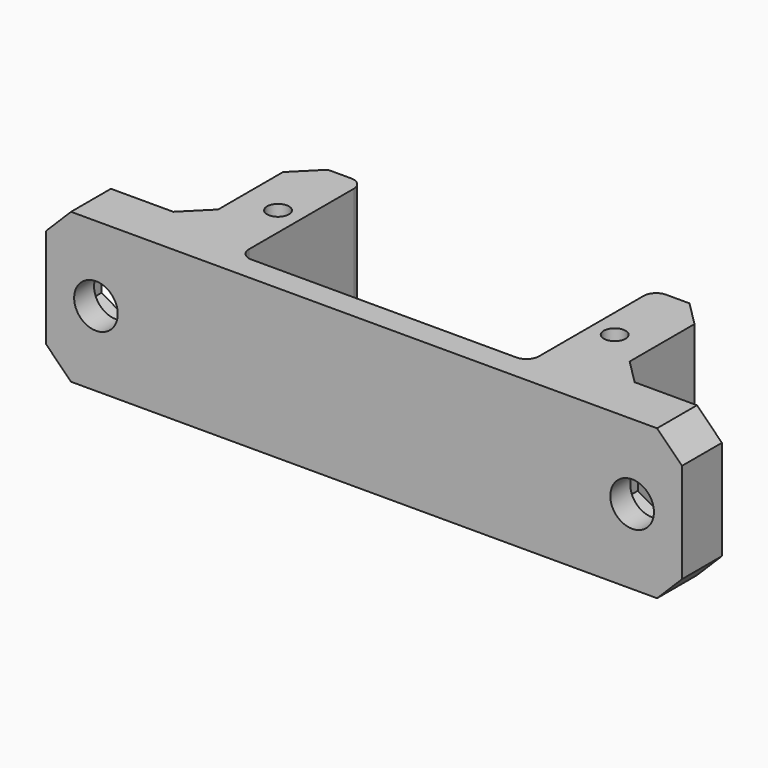
from build123d import *

# Parameters (mm, degrees)
F0_R     = 0.875
F1_DEPTH = 12
F2_SIZE  = 2
F3_R     = 1.75
F4_DEPTH = 4
F5_DEPTH = 2
F6_R     = 1


with BuildPart() as f1:
    # F0 (on Top) → F1 (new body)
    with BuildSketch(Plane.XY):
        Polygon((11.625, -5.25), (-11.625, -5.25), (-16.5, -5.25), (-16.5, -7.25), (16.5, -7.25), (16.5, -5.25), align=None)
        Polygon((-16.5, -5.25), (-16.5, -3.25), (-25.5, -3.25), (-25.5, -7.25), (-16.5, -7.25), align=None)
        Polygon((25.5, -3.25), (16.5, -3.25), (16.5, -5.25), (16.5, -7.25), (25.5, -7.25), align=None)
        Polygon((-11.625, 7.25), (-16.5, 7.25), (-16.5, -3.25), (-16.5, -5.25), (-11.625, -5.25), align=None)
        with Locations((-13.5, 1)):
            Circle(F0_R, mode=Mode.SUBTRACT)
        Polygon((16.5, 7.25), (11.625, 7.25), (11.625, -5.25), (16.5, -5.25), (16.5, -3.25), align=None)
        with Locations((13.5, 1)):
            Circle(F0_R, mode=Mode.SUBTRACT)
    extrude(amount=F1_DEPTH)

    # F2
    f2_edges = [f1.edges().sort_by_distance(p)[0] for p in [
        (-16.5, -3.25, 6),
        (16.5, -3.25, 6),
        (25.5, -5.25, 12),
        (25.5, -5.25, 0),
        (-25.5, -5.25, 12),
        (-25.5, -5.25, 0),
        (16.5, 7.25, 6),
        (-16.5, 7.25, 6),
    ]]
    chamfer(f2_edges, length=F2_SIZE)

    # F3 (on face) → F4 (cut, through all)
    with BuildSketch(Plane(origin=(0, -3.25, 0), x_dir=(-1, 0, 0), z_dir=(0, 1, 0))):
        with Locations((21.5, 6)):
            Circle(F3_R)
        with Locations((-21.5, 6)):
            Circle(F3_R)
    extrude(amount=-F4_DEPTH, mode=Mode.SUBTRACT)

    # F3 (on face) → F5 (cut)
    with BuildSketch(Plane(origin=(0, -3.25, 0), x_dir=(-1, 0, 0), z_dir=(0, 1, 0))):
        Polygon((-18.75, 4.4122867597), (-18.75, 7.5877132403), (-21.5, 9.1754264805), (-24.25, 7.5877132403), (-24.25, 4.4122867597), (-21.5, 2.8245735195), align=None)
        with Locations((-21.5, 6)):
            Circle(F3_R, mode=Mode.SUBTRACT)
        Polygon((18.75, 7.5877132403), (18.75, 4.4122867597), (21.5, 2.8245735195), (24.25, 4.4122867597), (24.25, 7.5877132403), (21.5, 9.1754264805), align=None)
        with Locations((21.5, 6)):
            Circle(F3_R, mode=Mode.SUBTRACT)
    extrude(amount=-F5_DEPTH, mode=Mode.SUBTRACT)

    # F6
    f6_edges = [f1.edges().sort_by_distance(p)[0] for p in [
        (11.625, -5.25, 6),
        (-11.625, -5.25, 6),
        (-11.625, 7.25, 6),
        (11.625, 7.25, 6),
    ]]
    fillet(f6_edges, radius=F6_R)


solid = f1.part
